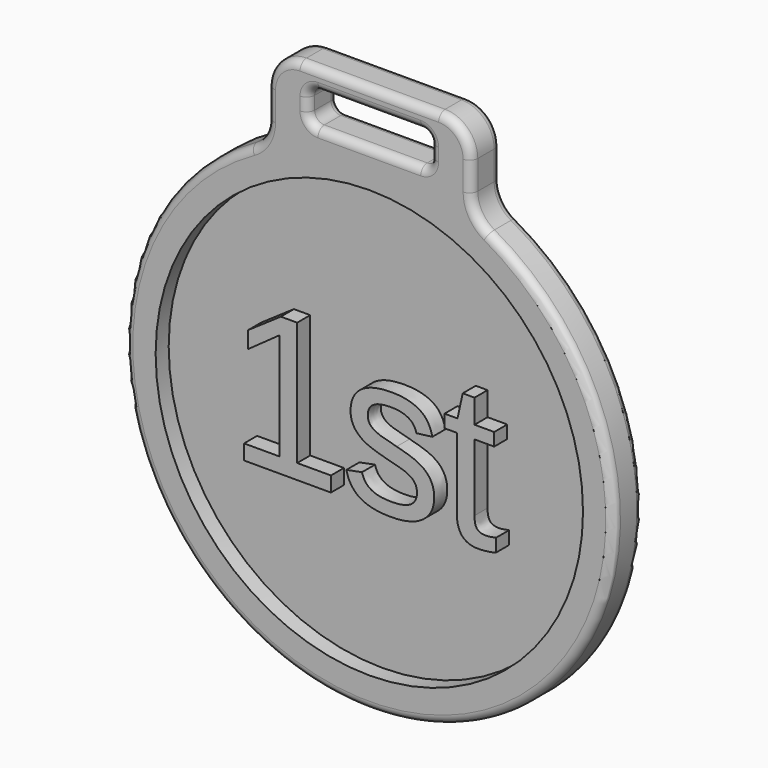
from build123d import *

# Parameters (mm, degrees)
F0_R         = 38.1
F1_DEPTH     = 3.175
F2_R         = 38.1
F2_R_2       = 33.274
F3_DEPTH     = 2.54
F4_TEXT_SIZE = 31.3701809805
F5_DEPTH     = 2.54
F6_W         = 19.05
F6_H         = 5.08
F7_DEPTH     = 5.715
F8_R         = 5.08
F9_R         = 1.524
F10_R        = 1.27


# Not quite as in the source:
# - Text() gives the source's letters only with a copy of the font that has no kerning and outlines rounded to 1/6400 em; it was checked with that copy


with BuildPart() as f1:
    # F0 (on Front) → F1 (new body)
    with BuildSketch(Plane.XZ):
        Circle(F0_R)
    extrude(amount=F1_DEPTH)

    # F2 (on face) → F3 (join)
    with BuildSketch(Plane.XZ.offset(3.175)):
        Circle(F2_R)
        Circle(F2_R_2, mode=Mode.SUBTRACT)
    extrude(amount=F3_DEPTH)

    # F4 (on face) → F5 (join, through all)
    with BuildSketch(Plane.XZ.offset(3.175)):
        with Locations((-21.8954060062, -10.1459566974)):
            Text('1st', F4_TEXT_SIZE, font='Arimo', text_align=(TextAlign.LEFT, TextAlign.BOTTOM))
    extrude(amount=F5_DEPTH)

    # F6 (on Front) → F7 (join, through all)
    with BuildSketch(Plane.XZ):
        with BuildLine():
            Line((15.875, 47.335160964), (-15.875, 47.335160964))
            Line((-15.875, 47.335160964), (-15.875, 34.635160964))
            ThreePointArc((-15.875, 34.635160964), (0, 38.1), (15.875, 34.635160964))
            Line((15.875, 34.635160964), (15.875, 47.335160964))
        make_face()
        with Locations((0, 41.620160964)):
            Rectangle(F6_W, F6_H, mode=Mode.SUBTRACT)
    extrude(amount=F7_DEPTH)

    # F8
    f8_edges = [f1.edges().sort_by_distance(p)[0] for p in [
        (15.875, -2.8575, 34.635161),
        (-15.875, -2.8575, 34.635161),
        (-15.875, -2.8575, 47.335161),
        (15.875, -2.8575, 47.335161),
    ]]
    fillet(f8_edges, radius=F8_R)

    # F9
    f9_edges = [f1.edges().sort_by_distance(p)[0] for p in [
        (-9.525, -2.8575, 39.080161),
        (-9.525, -2.8575, 44.160161),
        (9.525, -2.8575, 44.160161),
        (9.525, -2.8575, 39.080161),
    ]]
    fillet(f9_edges, radius=F9_R)

    # F10
    f10_edges = [f1.edges().sort_by_distance(p)[0] for p in [
        (0, -5.715, -38.1),
        (0, 0, -38.1),
        (0, -5.715, 39.080161),
        (0, 0, 39.080161),
    ]]
    fillet(f10_edges, radius=F10_R)


solid = f1.part
